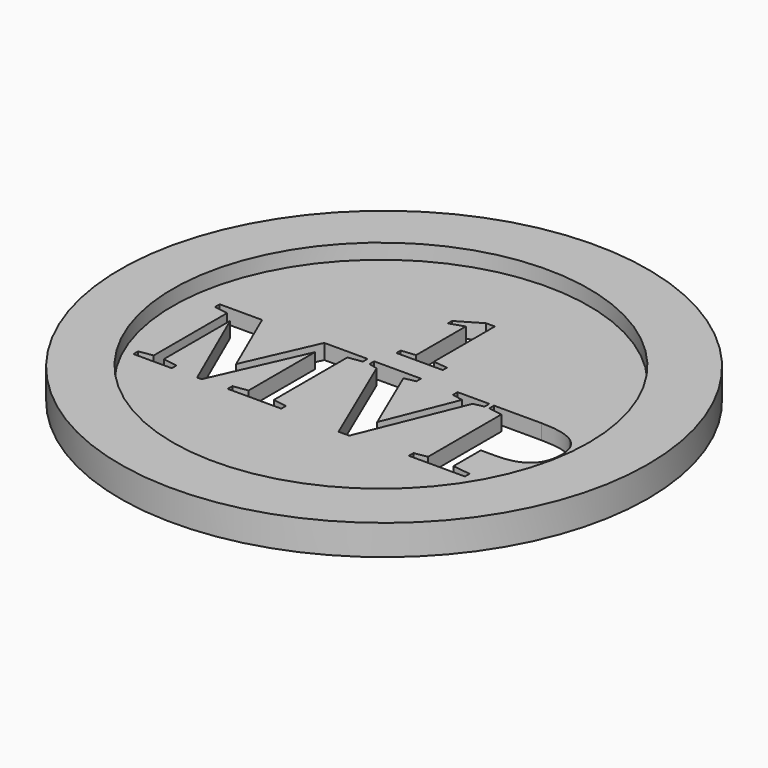
from build123d import *

# Parameters (mm, degrees)
F0_R     = 27.5956860517
F1_DEPTH = 2
F0_R_2   = 35
F2_DEPTH = 4


with BuildPart() as f1:
    # F0 (on Top) → F1 (new body)
    with BuildSketch(Plane.XY):
        Circle(F0_R)
        Polygon((-9.6259148038, 1.1057544772), (-15.0088759263, -10.9735011217), (-15.5956118662, -10.9735011217), (-20.8694128139, 1.1057544772), (-20.8694128139, -9.9057781613), (-18.952287243, -10.1957348758), (-18.952287243, -10.9735011217), (-24.0384691402, -10.9735011217), (-24.0384691402, -10.1957348758), (-22.2032137004, -9.9057781613), (-22.2032137004, 2.265581335), (-24.0384691402, 2.5453042831), (-24.0384691402, 3.3230705289), (-18.4201313906, 3.3230705289), (-14.3368585999, -6.0817607859), (-10.1683044226, 3.3230705289), (-4.4339839872, 3.3230705289), (-4.4339839872, 2.5453042831), (-6.2658281715, 2.265581335), (-6.2658281715, -9.9057781613), (-4.4339839872, -10.1957348758), (-4.4339839872, -10.9735011217), (-11.5430403747, -10.9735011217), (-11.5430403747, -10.1957348758), (-9.6259148038, -9.9057781613), align=None, mode=Mode.SUBTRACT)
        Polygon((7.508821393, 3.3230705289), (11.7183106359, 3.3230705289), (11.7183106359, 2.5453042831), (10.3640422166, 2.2553475686), (4.84121962, -11.3043929017), (3.4255486024, -11.3043929017), (-2.3838194532, 2.2553475686), (-3.5572913329, 2.5453042831), (-3.5572913329, 3.3230705289), (2.6580161229, 3.3230705289), (2.6580161229, 2.5453042831), (1.174119996, 2.2553475686), (5.1959901883, -7.1153711916), (8.948371199, 2.2553475686), (7.508821393, 2.5453042831), align=None, mode=Mode.SUBTRACT)
        with BuildLine():
            Line((19.4584492842, -5.3653971385), (17.5379124579, -5.3653971385))
            Line((17.5379124579, -5.3653971385), (17.5379124579, -9.9057781613))
            Line((17.5379124579, -9.9057781613), (19.9155575165, -10.1957348758))
            Line((19.9155575165, -10.1957348758), (19.9155575165, -10.9735011217))
            Line((19.9155575165, -10.9735011217), (12.475609349, -10.9735011217))
            Line((12.475609349, -10.9735011217), (12.475609349, -10.1957348758))
            Line((12.475609349, -10.1957348758), (14.1710033147, -9.9057781613))
            Line((14.1710033147, -9.9057781613), (14.1710033147, 2.265581335))
            Line((14.1710033147, 2.265581335), (12.3357478749, 2.5453042831))
            Line((12.3357478749, 2.5453042831), (12.3357478749, 3.3230705289))
            Line((12.3357478749, 3.3230705289), (18.6363367174, 3.3230705289))
            add(Edge.make_bspline(
                [(18.6363367174, 3.3230705289), (21.675765336, 3.3230705289), (23.178423368, 2.3048107729)],
                knots=[0, 0, 0, 1, 1, 1], degree=2))
            add(Edge.make_bspline(
                [(23.178423368, 2.3048107729), (24.6810814, 1.2865510168), (24.6810814, -0.8898299694)],
                knots=[0, 0, 0, 1, 1, 1], degree=2))
            add(Edge.make_bspline(
                [(24.6810814, -0.8898299694), (24.6810814, -5.3653971385), (19.4584492842, -5.3653971385)],
                knots=[0, 0, 0, 1, 1, 1], degree=2))
        make_face(mode=Mode.SUBTRACT)
        Polygon((1.3197273183, 17.2339269534), (1.3197273183, 7.1216629411), (3.216591065, 6.9262442858), (3.216591065, 6.2253427091), (-2.9221602911, 6.2253427091), (-2.9221602911, 6.9262442858), (-1.0331132906, 7.1216629411), (-1.0331132906, 15.3526966991), (-2.9143435449, 14.7351737486), (-2.9143435449, 15.4256529971), (0.1628488794, 17.2339269534), align=None, mode=Mode.SUBTRACT)
    extrude(amount=F1_DEPTH)

    # F0 (on Top) → F2 (join)
    with BuildSketch(Plane.XY):
        with Locations((0.418909197, 0)):
            Circle(F0_R_2)
        Circle(F0_R, mode=Mode.SUBTRACT)
    extrude(amount=F2_DEPTH)


solid = f1.part
